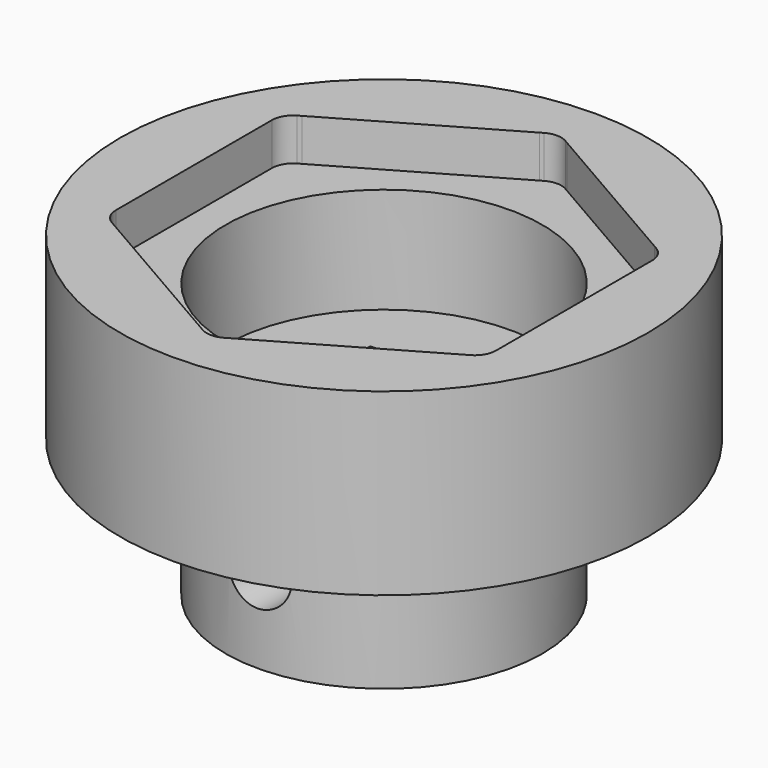
from build123d import *

# Parameters (mm, degrees)
F0_R           = 25
F1_DEPTH       = 30
F3_DEPTH       = 4
F4_R           = 15
F5_DEPTH       = 14
F6_W           = 13
F6_H           = 13
F7_DEPTH       = 30.001
F8_R           = 25
F8_R_2         = 15
F9_DEPTH       = 13
F10_R          = 3
F11_DEPTH      = 25.001
F11_DEPTH_BACK = 25.001
F12_S5_R       = 3
F12_T6_DEPTH   = 32
F13_R          = 0.15
F14_R          = 2


# Not quite as in the source:
# - a fillet or chamfer that OpenCascade refuses, or shapes differently, is made with other operations: its cross-section is extruded or revolved along the edge and cut away or added


with BuildPart() as f1:
    # F0 (on Top) → F1 (new body)
    with BuildSketch(Plane.XY):
        Circle(F0_R)
    extrude(amount=F1_DEPTH)

    # F2 (on face) → F3 (cut)
    with BuildSketch(Plane.XY.offset(30)):
        with BuildLine():
            Line((16.7009618943, 11.1423048454), (1.2990381057, 20.0346096908))
            ThreePointArc((1.2990381057, 20.0346096908), (0, 19.2846096908), (-1.2990381057, 20.0346096908))
            Line((-1.2990381057, 20.0346096908), (-16.7009618943, 11.1423048454))
            ThreePointArc((-16.7009618943, 11.1423048454), (-16.5511112606, 10.7805334131), (-16.5, 10.3923048454))
            ThreePointArc((-16.5, 10.3923048454), (-16.9393398282, 9.3316446736), (-18, 8.8923048454))
            Line((-18, 8.8923048454), (-18, -8.8923048454))
            ThreePointArc((-18, -8.8923048454), (-16.9393398282, -9.3316446736), (-16.5, -10.3923048454))
            ThreePointArc((-16.5, -10.3923048454), (-16.5511112606, -10.7805334131), (-16.7009618943, -11.1423048454))
            Line((-16.7009618943, -11.1423048454), (-1.2990381057, -20.0346096908))
            ThreePointArc((-1.2990381057, -20.0346096908), (0, -19.2846096908), (1.2990381057, -20.0346096908))
            Line((1.2990381057, -20.0346096908), (16.7009618943, -11.1423048454))
            ThreePointArc((16.7009618943, -11.1423048454), (16.7009618943, -9.6423048454), (18, -8.8923048454))
            Line((18, -8.8923048454), (18, 8.8923048454))
            ThreePointArc((18, 8.8923048454), (16.7009618943, 9.6423048454), (16.7009618943, 11.1423048454))
        make_face()
        with BuildLine():
            ThreePointArc((-16.5, 10.3923048454), (-16.5511112606, 10.7805334131), (-16.7009618943, 11.1423048454))
            Line((-16.7009618943, 11.1423048454), (-18, 10.3923048454))
            Line((-18, 10.3923048454), (-18, 8.8923048454))
            ThreePointArc((-18, 8.8923048454), (-16.9393398282, 9.3316446736), (-16.5, 10.3923048454))
        make_face()
        with BuildLine():
            ThreePointArc((-16.5, -10.3923048454), (-16.9393398282, -9.3316446736), (-18, -8.8923048454))
            Line((-18, -8.8923048454), (-18, -10.3923048454))
            Line((-18, -10.3923048454), (-16.7009618943, -11.1423048454))
            ThreePointArc((-16.7009618943, -11.1423048454), (-16.5511112606, -10.7805334131), (-16.5, -10.3923048454))
        make_face()
        with BuildLine():
            Line((0, -20.7846096908), (1.2990381057, -20.0346096908))
            ThreePointArc((1.2990381057, -20.0346096908), (0, -19.2846096908), (-1.2990381057, -20.0346096908))
            Line((-1.2990381057, -20.0346096908), (0, -20.7846096908))
        make_face()
        with BuildLine():
            Line((18, -10.3923048454), (18, -8.8923048454))
            ThreePointArc((18, -8.8923048454), (16.7009618943, -9.6423048454), (16.7009618943, -11.1423048454))
            Line((16.7009618943, -11.1423048454), (18, -10.3923048454))
        make_face()
        with BuildLine():
            Line((18, 10.3923048454), (16.7009618943, 11.1423048454))
            ThreePointArc((16.7009618943, 11.1423048454), (16.7009618943, 9.6423048454), (18, 8.8923048454))
            Line((18, 8.8923048454), (18, 10.3923048454))
        make_face()
        with BuildLine():
            Line((1.2990381057, 20.0346096908), (0, 20.7846096908))
            Line((0, 20.7846096908), (-1.2990381057, 20.0346096908))
            ThreePointArc((-1.2990381057, 20.0346096908), (0, 19.2846096908), (1.2990381057, 20.0346096908))
        make_face()
    extrude(amount=-F3_DEPTH, mode=Mode.SUBTRACT)

    # F4 (on face) → F5 (cut)
    with BuildSketch(Plane.XY.offset(30)):
        Circle(F4_R)
    extrude(amount=-F5_DEPTH, mode=Mode.SUBTRACT)

    # F6 (on face) → F7 (cut, through all)
    with BuildSketch(Plane(origin=(0, 0, 0), x_dir=(1, 0, 0), z_dir=(0, 0, -1))):
        Rectangle(F6_W, F6_H)
    extrude(amount=-F7_DEPTH, mode=Mode.SUBTRACT)

    # F8 (on face) → F9 (cut)
    with BuildSketch(Plane(origin=(0, 0, 0), x_dir=(1, 0, 0), z_dir=(0, 0, -1))):
        Circle(F8_R)
        Circle(F8_R_2, mode=Mode.SUBTRACT)
    extrude(amount=-F9_DEPTH, mode=Mode.SUBTRACT)

    # F10 (on Front) → F11 (cut, two sides)
    with BuildSketch(Plane.XZ) as f11_sk:
        with Locations((0, 8)):
            Circle(F10_R)
    extrude(amount=-F11_DEPTH, mode=Mode.SUBTRACT)
    extrude(f11_sk.sketch, amount=F11_DEPTH_BACK, mode=Mode.SUBTRACT)

    # F12: fillet of radius 5 on 1 edges, made by hand


with BuildPart() as f12_tool2:
    # F12_s3 → F12_t4 (revolve)
    with BuildSketch(Plane.XZ):
        with BuildLine():
            ThreePointArc((20, 13), (16.4644660941, 11.5355339059), (15, 8))
            Line((15, 8), (15, 13))
            Line((15, 13), (20, 13))
        make_face()
    revolve(axis=Axis((0, 0, 13), (0, 0, -1)))

    # F12_s5 → F12_t6 (cut, symmetric)
    with BuildSketch(Plane.XZ):
        with Locations((0, 8)):
            Circle(F12_S5_R)
    extrude(amount=F12_T6_DEPTH, both=True, mode=Mode.SUBTRACT)


with BuildPart() as f1_1:
    add(f1.part)

    # F12_t1: union F12_tool2
    add(f12_tool2.part)

    # F13
    f13_edges = [f1_1.edges().sort_by_distance(p)[0] for p in [
        (-6.5, -6.5, 8),
        (-6.5, 6.5, 8),
        (6.5, 6.5, 8),
        (6.5, -6.5, 8),
    ]]
    fillet(f13_edges, radius=F13_R)

    # F14
    f14_edges = [f1_1.edges().sort_by_distance(p)[0] for p in [
        (-18, -10.392305, 28),
        (-18, 10.392305, 28),
        (0, -20.78461, 28),
        (18, -10.392305, 28),
        (18, 10.392305, 28),
        (0, 20.78461, 28),
    ]]
    fillet(f14_edges, radius=F14_R)


solid = f1_1.part
